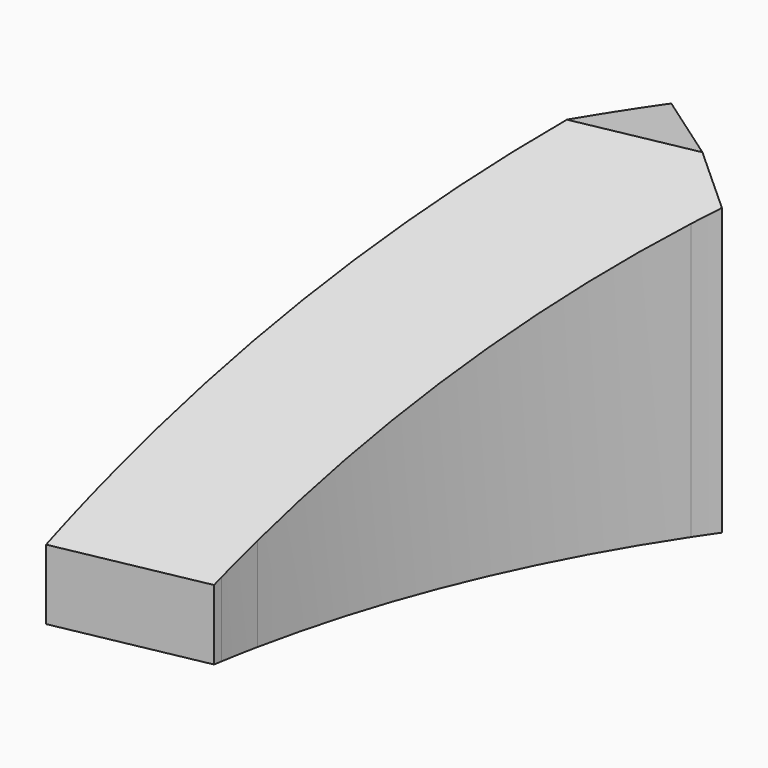
from build123d import *

# Parameters (mm, degrees)
F0_R        = 1.5
F1_DEPTH    = 22
F2_T1_DEPTH = 165.8159550338
F3_DEPTH    = 8


# Not quite as in the source:
# - a fillet or chamfer that OpenCascade refuses, or shapes differently, is made with other operations: its cross-section is extruded or revolved along the edge and cut away or added


with BuildPart() as f1:
    # F0 (on Top) → F1 (new body)
    with BuildSketch(Plane.XY):
        with BuildLine():
            ThreePointArc((-71.5091042417, 11.9456272565), (-71.2779515077, 13.2553245479), (-71.0228136012, 14.5605613962))
            Line((-71.0228136012, 14.5605613962), (-78.4331581972, 13.1022935094))
            Line((-78.4331581972, 13.1022935094), (-71.5091042417, 11.9456272565))
        make_face()
        with BuildLine():
            ThreePointArc((-71.0228136012, 14.5605613962), (-66.9578457789, 27.8010231583), (-60.4491628751, 40.0268498348))
            Line((-60.4491628751, 40.0268498348), (-68.7869784441, 45.5477946397))
            ThreePointArc((-68.7869784441, 45.5477946397), (-76.7608906967, 30.2326918988), (-81.3724289647, 13.5932999815))
            Line((-81.3724289647, 13.5932999815), (-78.4331581972, 13.1022935094))
            Line((-78.4331581972, 13.1022935094), (-71.0228136012, 14.5605613962))
        make_face()
        with Locations((-74.7222680365, 20.5628952117)):
            Circle(F0_R, mode=Mode.SUBTRACT)
        with Locations((-67.9969340878, 37.184229919)):
            Circle(F0_R, mode=Mode.SUBTRACT)
        with BuildLine():
            ThreePointArc((-60.4491628751, 40.0268498348), (-59.9428373222, 40.7811997588), (-59.4270987125, 41.5291456523))
            Line((-59.4270987125, 41.5291456523), (-67.6239399142, 47.2573036734))
            ThreePointArc((-67.6239399142, 47.2573036734), (-68.2108148839, 46.4061928289), (-68.7869784441, 45.5477946397))
            Line((-68.7869784441, 45.5477946397), (-60.4491628751, 40.0268498348))
        make_face()
        with BuildLine():
            ThreePointArc((-71.5997882434, 11.3894830218), (-71.554986557, 11.667643242), (-71.5091042417, 11.9456272565))
            Line((-71.5091042417, 11.9456272565), (-78.4331581972, 13.1022935094))
            Line((-78.4331581972, 13.1022935094), (-81.5492033125, 12.4890928052))
            ThreePointArc((-81.5492033125, 12.4890928052), (-81.7739574871, 10.9210748966), (-81.9685648448, 9.3490308206))
            Line((-81.9685648448, 9.3490308206), (-71.5997882434, 11.3894830219))
        make_face()
        with BuildLine():
            Line((-81.5492033125, 12.4890928052), (-78.4331581972, 13.1022935094))
            Line((-78.4331581972, 13.1022935094), (-81.3724289647, 13.5932999815))
            ThreePointArc((-81.3724289647, 13.5932999815), (-81.462687068, 13.0414959135), (-81.5492033125, 12.4890928052))
        make_face()
        with Locations((-67.9969340878, 37.184229919)):
            Circle(F0_R)
        with Locations((-74.7222680365, 20.5628952117)):
            Circle(F0_R)
    extrude(amount=F1_DEPTH)

    # F2: chamfer of 17 x 30 on 1 edges, made by hand

    # F2_s2 → F2_t1 (cut)
    with BuildSketch(Plane(origin=(-153.3048702431, -30.1685793773, 0), x_dir=(0, 0, 1), z_dir=(0.9811820369, 0.1930849823, 0))):
        Polygon((5, -25), (22, -55), (22, -25), align=None)
    extrude(amount=F2_T1_DEPTH, mode=Mode.SUBTRACT)

    # F0 (on Top) → F3 (cut)
    with BuildSketch(Plane.XY):
        with Locations((-67.9969340878, 37.184229919)):
            Circle(F0_R)
        with Locations((-74.7222680365, 20.5628952117)):
            Circle(F0_R)
    extrude(amount=F3_DEPTH, mode=Mode.SUBTRACT)


solid = f1.part
